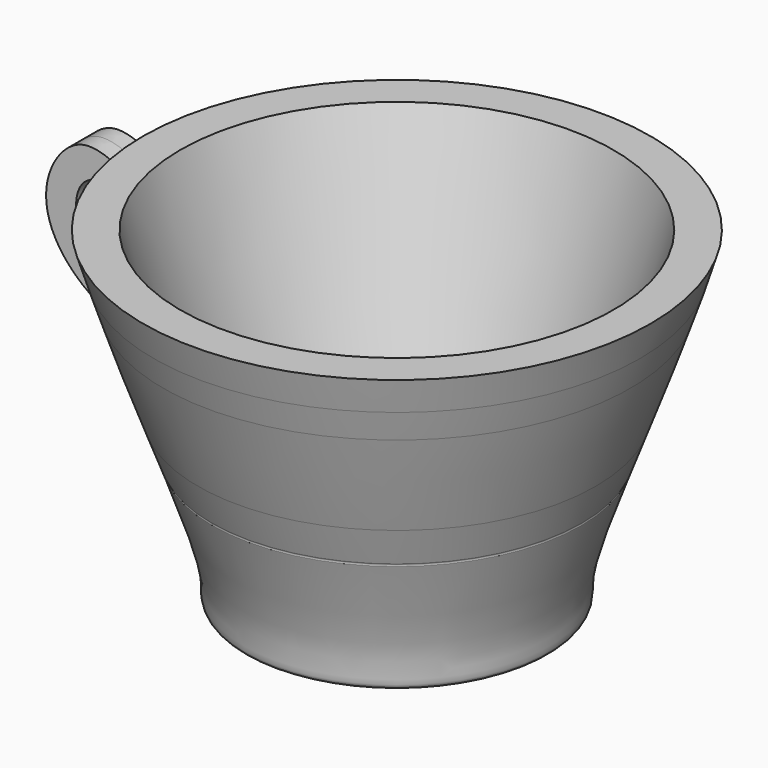
from build123d import *

# Parameters (mm, degrees)
F1_DEPTH = 6.35


with BuildPart() as f1:
    # F0 (on Front) → F1 (new body, symmetric)
    with BuildSketch(Plane.XZ):
        with BuildLine():
            add(Edge.make_bspline(
                [(-26.779282031, 30.8305839929), (-25.6599872306, 27.3359164201), (-24.5269169087, 23.8945397492), (-23.388681933, 20.5122753915)],
                knots=[0.0572413722, 0.0572413722, 0.0572413722, 0.0572413722, 0.1081291612, 0.1081291612, 0.1081291612, 0.1081291612], degree=3))
            add(Edge.make_bspline(
                [(-26.779282031, 30.8305839929), (-33.9641073682, 34.8686155193), (-47.7904028814, 43.0881960424), (-64.5885629334, 19.6560020505), (-50.1366297488, -11.4458780792), (-9.2230358971, -24.1099512444), (-6.4222046506, -26.6422513876)],
                knots=[0, 0, 0, 0, 0.206318069, 0.4087967984, 0.6632998285, 0.9539101751, 0.9539101751, 0.9539101751, 0.9539101751], degree=3))
            add(Edge.make_bspline(
                [(-11.1529605838, -13.8355021779), (-9.5017867072, -18.3061029042), (-7.914064356, -22.5823231964), (-6.4222046506, -26.6422513876)],
                knots=[0.2936194992, 0.2936194992, 0.2936194992, 0.2936194992, 0.3727777079, 0.3727777079, 0.3727777079, 0.3727777079], degree=3))
            add(Edge.make_bspline(
                [(-23.388681933, 20.5122753915), (-31.3587647344, 24.7259859161), (-44.4741122772, 32.263043577), (-51.7309465833, 16.3828269272), (-39.4091940553, -2.9788718203), (-21.3549569349, -10.0574184983), (-11.1529605838, -13.8355021779)],
                knots=[0, 0, 0, 0, 0.2571458127, 0.4422215918, 0.6928586951, 1, 1, 1, 1], degree=3))
        make_face()
    extrude(amount=F1_DEPTH, both=True)

    # F0 (on Front) → F2 (revolve)
    with BuildSketch(Plane.XZ):
        with BuildLine():
            Line((-17.4031369388, 42.8175656639), (-30.4918682477, 42.8175656639))
            add(Edge.make_bspline(
                [(-30.4918682477, 42.8175656639), (-29.2799400842, 38.7599998745), (-28.0383261293, 34.761577491), (-26.779282031, 30.8305839929)],
                knots=[0, 0, 0, 0, 0.0572413722, 0.0572413722, 0.0572413722, 0.0572413722], degree=3))
            add(Edge.make_bspline(
                [(-26.779282031, 30.8305839929), (-25.6599872306, 27.3359164201), (-24.5269169087, 23.8945397492), (-23.388681933, 20.5122753915)],
                knots=[0.0572413722, 0.0572413722, 0.0572413722, 0.0572413722, 0.1081291612, 0.1081291612, 0.1081291612, 0.1081291612], degree=3))
            add(Edge.make_bspline(
                [(-23.388681933, 20.5122753915), (-19.2397182058, 8.1836328569), (-15.0221335422, -3.3596051914), (-11.1529605838, -13.8355021779)],
                knots=[0.1081291612, 0.1081291612, 0.1081291612, 0.1081291612, 0.2936194992, 0.2936194992, 0.2936194992, 0.2936194992], degree=3))
            add(Edge.make_bspline(
                [(-11.1529605838, -13.8355021779), (-9.5017867072, -18.3061029042), (-7.914064356, -22.5823231964), (-6.4222046506, -26.6422513876)],
                knots=[0.2936194992, 0.2936194992, 0.2936194992, 0.2936194992, 0.3727777079, 0.3727777079, 0.3727777079, 0.3727777079], degree=3))
            add(Edge.make_bspline(
                [(-6.4222046506, -26.6422513876), (-5.9780022219, -27.0438656852), (-6.0119811368, -27.339355921), (-6.0560090254, -27.6397535643)],
                knots=[0.9539101751, 0.9539101751, 0.9539101751, 0.9539101751, 1, 1, 1, 1], degree=3))
            add(Edge.make_bspline(
                [(-6.0560090254, -27.6397535643), (0.0825960797, -44.3776523907), (8.441969007, -68.8198420623), (2.4540492736, -74.2481329269), (23.0473924894, -71.2587758899)],
                knots=[0.3792892362, 0.3792892362, 0.3792892362, 0.3792892362, 0.7085331873, 1, 1, 1, 1], degree=3))
            Line((23.0473924894, -71.2587758899), (58.7943717837, -71.2587758899))
            Line((58.7943717837, -71.2587758899), (58.7943717837, -63.262745738))
            Line((58.7943717837, -63.262745738), (14.1106499359, -63.262745738))
            Line((14.1106499359, -63.262745738), (-17.4031369388, 42.8175656639))
        make_face()
    revolve(axis=Axis((58.7943717837, 0, -67.260760814), (0, 0, -1)))


solid = f1.part
